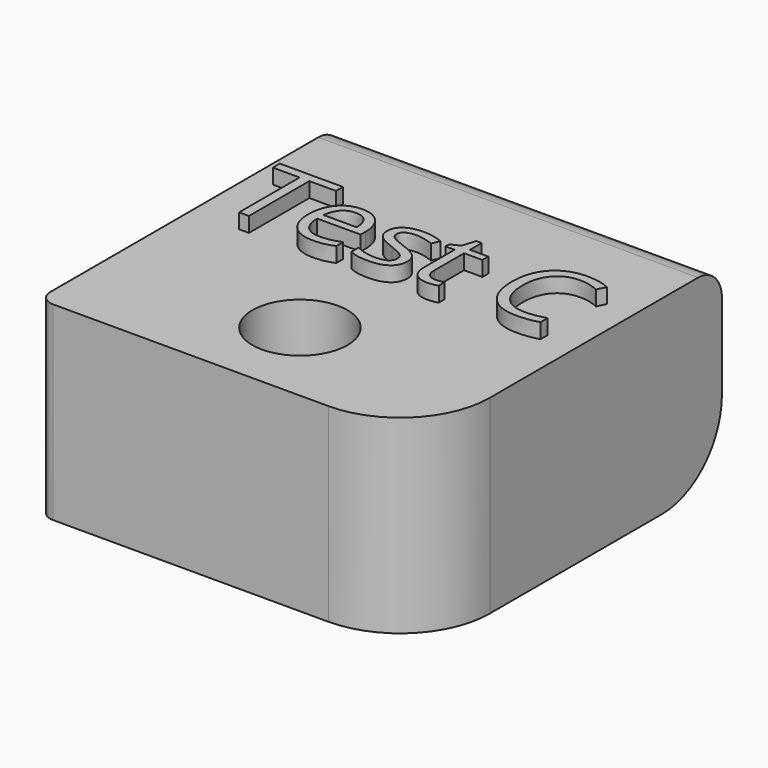
from build123d import *

# Parameters (mm, degrees)
F0_W         = 25.4
F0_H         = 25.4
F1_DEPTH     = 12.7
F2_R         = 3.175
F3_DEPTH     = 12.701
F4_R         = 6
F5_R         = 1
F6_R         = 2
F7_R         = 5
F8_TEXT_SIZE = 7.8871225317
F9_DEPTH     = 1


# Not quite as in the source:
# - Text() gives the source's letters only with a copy of the font that has no kerning and outlines rounded to 1/6400 em; it was checked with that copy


with BuildPart() as f1:
    # F0 (on Top) → F1 (new body)
    with BuildSketch(Plane.XY):
        Rectangle(F0_W, F0_H)
    extrude(amount=F1_DEPTH)

    # F2 (on face) → F3 (cut, through all)
    with BuildSketch(Plane.XY.offset(12.7)):
        with Locations((0, -6.7)):
            Circle(F2_R)
    extrude(amount=-F3_DEPTH, mode=Mode.SUBTRACT)

    # F4
    f4_edges = [f1.edges().sort_by_distance(p)[0] for p in [
        (12.7, -12.7, 6.35),
    ]]
    fillet(f4_edges, radius=F4_R)

    # F5
    f5_edges = [f1.edges().sort_by_distance(p)[0] for p in [
        (-12.7, -12.7, 6.35),
    ]]
    fillet(f5_edges, radius=F5_R)

    # F6
    f6_edges = [f1.edges().sort_by_distance(p)[0] for p in [
        (0, 12.7, 12.7),
    ]]
    fillet(f6_edges, radius=F6_R)

    # F7
    f7_edges = [f1.edges().sort_by_distance(p)[0] for p in [
        (0, 12.7, 0),
    ]]
    fillet(f7_edges, radius=F7_R)

    # F8 (on face) → F9 (join)
    with BuildSketch(Plane.XY.offset(12.7)):
        with Locations((-11.277503334, 0)):
            Text('Test C', F8_TEXT_SIZE, font='Open Sans', text_align=(TextAlign.LEFT, TextAlign.BOTTOM))
    extrude(amount=F9_DEPTH)


solid = f1.part
